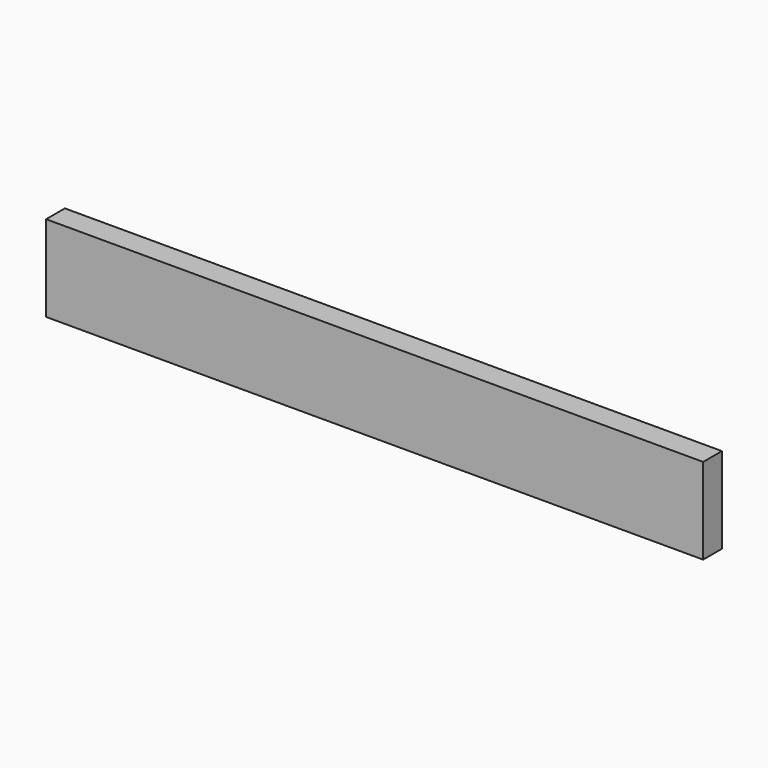
from build123d import *

# Parameters (mm, degrees)
F1_W     = 38.1
F1_H     = 139.7
F2_DEPTH = 1066.8


# Not quite as in the source:
# - a variable given as a bare number and used for a length is read in inches; the dataset says mm whatever the document's units were


with BuildPart() as f2:
    # F1 (on Right) → F2 (new body)
    with BuildSketch(Plane.YZ):
        with Locations((-30.8593586087, 51.4001077512)):
            Rectangle(F1_W, F1_H)
    extrude(amount=F2_DEPTH)


solid = f2.part
